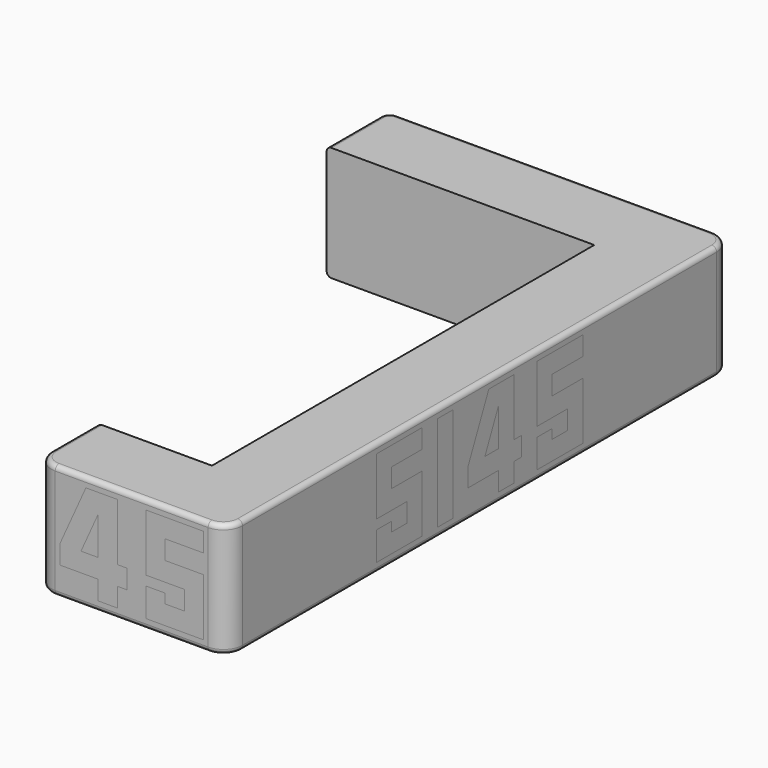
from build123d import *

# Parameters (mm, degrees)
F1_DEPTH  = 152.4
F2_R      = 25.4
F3_W      = 25.4
F3_H      = 127
F4_DEPTH  = 25.4
F5_DEPTH  = 25.4
F7_DEPTH  = 25.4
F8_DEPTH  = 25.4
F9_W      = 25.4
F9_H      = 127
F10_DEPTH = 25.4
F11_DEPTH = 25.4
F12_R     = 12.69999
F13_R     = 6.35


# Not quite as in the source:
# - a fillet or chamfer is up to 0.001 mm smaller than in the source, because OpenCascade refuses the exact size


with BuildPart() as f1:
    # F0 (on Top) → F1 (new body)
    with BuildSketch(Plane.XY):
        Polygon((-261.3841307829, 381.0432040095), (-261.3841307829, 279.4432040095), (94.2158692171, 279.4432040095), (94.2158692171, -355.5567959905), (-58.1841307829, -355.5567959905), (-58.1841307829, -457.1567959905), (195.8158692171, -457.1567959905), (195.8158692171, 381.0432040095), align=None)
    extrude(amount=F1_DEPTH)

    # F2
    f2_edges = [f1.edges().sort_by_distance(p)[0] for p in [
        (195.815869, -457.156796, 76.2),
        (-58.184131, -457.156796, 76.2),
        (195.815869, 381.043204, 76.2),
    ]]
    fillet(f2_edges, radius=F2_R)

    # F3 (on face) → F4 (cut)
    with BuildSketch(Plane.YZ.offset(195.8158692171)):
        Polygon((-133.3067959905, 114.3), (-133.3067959905, 139.7), (-209.5067959905, 139.7), (-209.5067959905, 63.5), (-158.7067959905, 63.5), (-158.7067959905, 38.1), (-184.1067959905, 38.1), (-184.1067959905, 50.8), (-209.5067959905, 50.8), (-209.5067959905, 12.7), (-133.3067959905, 12.7), (-133.3067959905, 88.9), (-184.1067959905, 88.9), (-184.1067959905, 114.3), align=None)
        with Locations((-95.2067959905, 76.2)):
            Rectangle(F3_W, F3_H)
        Polygon((19.0932040095, 63.5), (19.0932040095, 139.7), (-22.7088792915, 139.7), (-57.1067959905, 63.5), (-57.1067959905, 38.1), (-6.3067959905, 38.1), (-6.3067959905, 12.7), (19.0932040095, 12.7), (19.0932040095, 38.1), (31.7932040095, 38.1), (31.7932040095, 63.5), align=None)
        Polygon((-6.3067959905, 114.3), (-6.3067959905, 63.5), (-29.2387404565, 63.5), align=None, mode=Mode.SUBTRACT)
        Polygon((133.3932040095, 114.3), (133.3932040095, 139.7), (57.1932040095, 139.7), (57.1932040095, 63.5), (107.9932040095, 63.5), (107.9932040095, 38.1), (82.5932040095, 38.1), (82.5932040095, 50.8), (57.1932040095, 50.8), (57.1932040095, 12.7), (133.3932040095, 12.7), (133.3932040095, 88.9), (82.5932040095, 88.9), (82.5932040095, 114.3), align=None)
    extrude(amount=-F4_DEPTH, mode=Mode.SUBTRACT)


with BuildPart() as f5:
    # F5 (new): a face of the model
    f5_faces = [f1.part.faces().sort_by_distance(p)[0] for p in [
        (170.4158692171, -172.5111438166, 74.8195652174),
    ]]
    extrude(f5_faces, amount=F5_DEPTH)


with BuildPart() as f5b:
    # F5#2 (new): a face of the model
    f5_2_faces = [f1.part.faces().sort_by_distance(p)[0] for p in [
        (170.4158692171, -95.2067959905, 76.2),
    ]]
    extrude(f5_2_faces, amount=F5_DEPTH)


with BuildPart() as f5c:
    # F5#3 (new): a face of the model
    f5_3_faces = [f1.part.faces().sort_by_distance(p)[0] for p in [
        (170.4158692171, 25.4432040095, 61.9497674368),
    ]]
    extrude(f5_3_faces, amount=F5_DEPTH)


with BuildPart() as f5d:
    # F5#4 (new): a face of the model
    f5_4_faces = [f1.part.faces().sort_by_distance(p)[0] for p in [
        (170.4158692171, 94.1888561834, 74.8195652174),
    ]]
    extrude(f5_4_faces, amount=F5_DEPTH)


with BuildPart() as f1_1:
    add(f1.part)

    # F6 (on face) → F7 (cut)
    with BuildSketch(Plane.XZ.offset(457.1567959905)):
        Polygon((49.7658692171, 139.7), (7.9637859161, 139.7), (-26.4341307829, 63.5), (-26.4341307829, 38.1), (24.3658692171, 38.1), (24.3658692171, 12.7), (49.7658692171, 12.7), (49.7658692171, 38.1), (62.4658692171, 38.1), (62.4658692171, 63.5), (49.7658692171, 63.5), align=None)
        Polygon((24.3658692171, 114.3), (24.3658692171, 63.5), (1.4339247512, 63.5), align=None, mode=Mode.SUBTRACT)
        Polygon((164.0658692171, 114.3), (164.0658692171, 139.7), (87.8658692171, 139.7), (87.8658692171, 63.5), (138.6658692171, 63.5), (138.6658692171, 38.1), (113.2658692171, 38.1), (113.2658692171, 50.8), (87.8658692171, 50.8), (87.8658692171, 12.7), (164.0658692171, 12.7), (164.0658692171, 88.9), (113.2658692171, 88.9), (113.2658692171, 114.3), align=None)
    extrude(amount=-F7_DEPTH, mode=Mode.SUBTRACT)


with BuildPart() as f8:
    # F8 (new): a face of the model
    f8_faces = [f1_1.part.faces().sort_by_distance(p)[0] for p in [
        (48.2156366539, -431.7567959905, 101.6),
    ]]
    extrude(f8_faces, amount=F8_DEPTH)


with BuildPart() as f8b:
    # F8#2 (new): a face of the model
    f8_2_faces = [f1_1.part.faces().sort_by_distance(p)[0] for p in [
        (124.8615213911, -431.7567959905, 74.8195652174),
    ]]
    extrude(f8_2_faces, amount=F8_DEPTH)


with BuildPart() as f1_2:
    add(f1_1.part)

    # F9 (on face) → F10 (cut)
    with BuildSketch(Plane(origin=(0, 381.0432040095, 0), x_dir=(-1, 0, 0), z_dir=(0, 1, 0))):
        Polygon((197.8841307829, 114.3), (197.8841307829, 139.7), (121.6841307829, 139.7), (121.6841307829, 63.5), (172.4841307829, 63.5), (172.4841307829, 38.1), (147.0841307829, 38.1), (147.0841307829, 50.8), (121.6841307829, 50.8), (121.6841307829, 12.7), (197.8841307829, 12.7), (197.8841307829, 88.9), (147.0841307829, 88.9), (147.0841307829, 114.3), align=None)
        with Locations((235.9841307829, 76.2)):
            Rectangle(F9_W, F9_H)
    extrude(amount=-F10_DEPTH, mode=Mode.SUBTRACT)


with BuildPart() as f11:
    # F11 (new): a face of the model
    f11_faces = [f1_2.part.faces().sort_by_distance(p)[0] for p in [
        (-158.6797829568, 355.6432040095, 74.8195652174),
    ]]
    extrude(f11_faces, amount=F11_DEPTH)


with BuildPart() as f11b:
    # F11#2 (new): a face of the model
    f11_2_faces = [f1_2.part.faces().sort_by_distance(p)[0] for p in [
        (-235.9841307829, 355.6432040095, 76.2),
    ]]
    extrude(f11_2_faces, amount=F11_DEPTH)


with BuildPart() as f1_3:
    add(f1_2.part)

    # F12 (radius 12.7 in the source; OpenCascade refuses exactly that, so slightly less here)
    f12_edges = [f1_3.edges().sort_by_distance(p)[0] for p in [
        (-261.384131, 381.043204, 76.2),
    ]]
    fillet(f12_edges, radius=F12_R)

    # F13
    f13_edges = [f1_3.edges().sort_by_distance(p)[0] for p in [
        (195.815869, -38.056796, 152.4),
        (195.815869, -38.056796, 0),
    ]]
    fillet(f13_edges, radius=F13_R)


solid = Compound([f5.part, f5b.part, f5c.part, f5d.part, f8.part, f8b.part, f11.part, f11b.part, f1_3.part])
